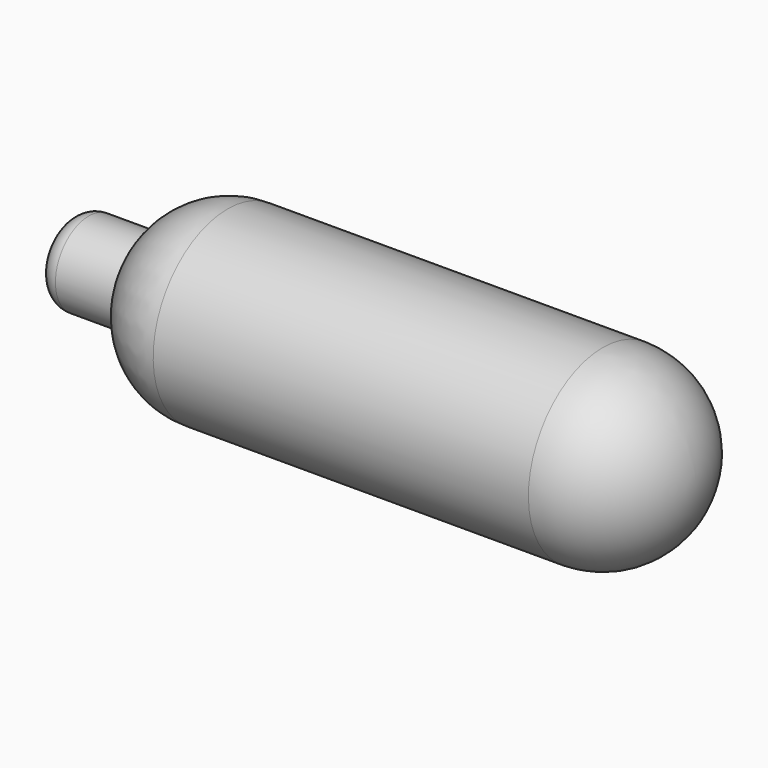
from build123d import *

# Parameters (mm, degrees)
F2_R = 9.5
F4_R = 2


# Not quite as in the source:
# - a fillet or chamfer that OpenCascade refuses, or shapes differently, is made with other operations: its cross-section is extruded or revolved along the edge and cut away or added


with BuildPart() as f1:
    # F0 (on Front) → F1 (revolve)
    with BuildSketch(Plane.XZ):
        Polygon((0, 4.25), (0, 0), (64, 0), (64, 9.5), (8, 9.5), (8, 4.25), align=None)
    revolve(axis=Axis((32, 0, 0), (1, 0, 0)))

    # F2
    f2_edges = [f1.edges().sort_by_distance(p)[0] for p in [
        (64, 0, -9.5),
    ]]
    fillet(f2_edges, radius=F2_R)

    # F3: fillet of radius 9 on 1 edges, made by hand

    # F3_s1 → F3_t2 (revolve, cut)
    with BuildSketch(Plane.XZ):
        with BuildLine():
            ThreePointArc((16.181534086, 9.5), (11.3209785622, 8.0746287038), (8, 4.25))
            Line((8, 4.25), (8, 9.5))
            Line((8, 9.5), (16.181534086, 9.5))
        make_face()
    revolve(axis=Axis((8, 0, 0), (1, 0, 0)), mode=Mode.SUBTRACT)

    # F4
    f4_edges = [f1.edges().sort_by_distance(p)[0] for p in [
        (0, 0, -4.25),
    ]]
    fillet(f4_edges, radius=F4_R)


solid = f1.part
